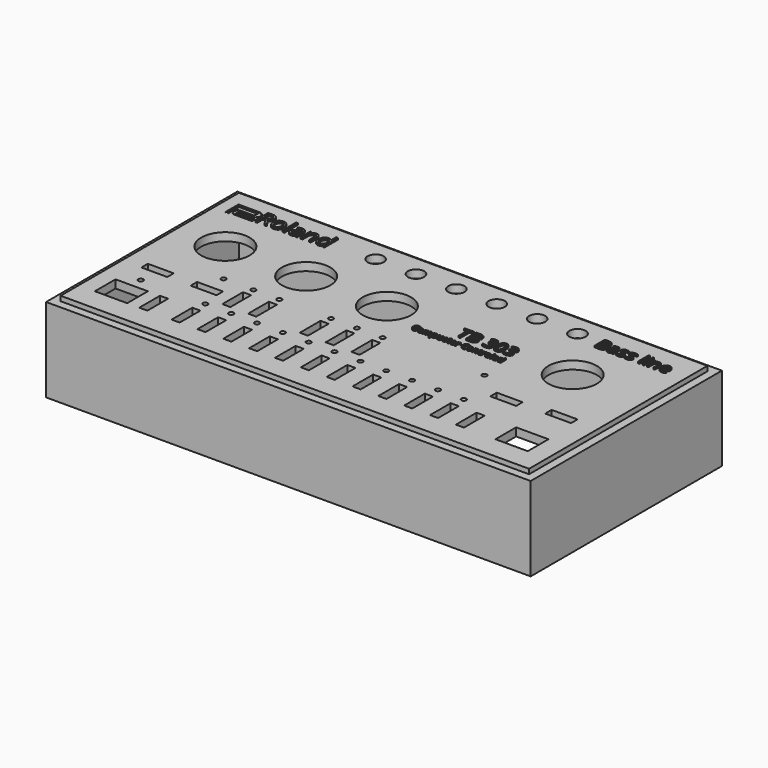
from build123d import *

# Parameters (mm, degrees)
F6_START       = 50
F0_W           = 290
F0_H           = 138
F6_DEPTH       = 5
F7_START       = 50
F4_W           = 5
F4_H           = 16
F4_W_2         = 20
F4_W_3         = 16
F4_H_2         = 5
F4_R           = 1.5
F3_R           = 15
F2_R           = 5
F7_DEPTH       = 5
F0_W_2         = 300
F0_H_2         = 148
F8_DEPTH       = 52
F9_START       = 55
F5_TEXT_SIZE   = 11.1111111111
F9_DEPTH       = 1
F10_START      = 55
F5_TEXT_SIZE_2 = 5.5555555556
F10_DEPTH      = 1
F11_START      = 55
F5_TEXT_SIZE_3 = 13.8888888889
F11_DEPTH      = 1
F12_START      = 55
F12_DEPTH      = 1
F15_W          = 0.5
F15_H          = 0.5


# Not quite as in the source:
# - a feature names something its author has since deleted; it is built from what else it names
# - Text() gives the source's letters only with a copy of the font that has no kerning and outlines rounded to 1/6400 em; it was checked with that copy


with BuildPart() as f6:
    # F0 (on Top) → F6 (new body)
    with BuildSketch(Plane.XY.offset(F6_START)):
        with Locations((150, 74)):
            Rectangle(F0_W, F0_H)
    extrude(amount=F6_DEPTH)

    # F4 (on Top) + F3 (on Top) + F2 (on Top) → F7 (cut)
    with BuildSketch(Plane.XY.offset(F7_START)):
        with Locations((161, 27)):
            Rectangle(F4_W, F4_H)
        with Locations((97, 27)):
            Rectangle(F4_W, F4_H)
        with Locations((241, 27)):
            Rectangle(F4_W, F4_H)
        with Locations((129, 27)):
            Rectangle(F4_W, F4_H)
        with Locations((113, 27)):
            Rectangle(F4_W, F4_H)
        with Locations((145, 27)):
            Rectangle(F4_W, F4_H)
        with Locations((177, 27)):
            Rectangle(F4_W, F4_H)
        with Locations((225, 27)):
            Rectangle(F4_W, F4_H)
        with Locations((25, 27)):
            Rectangle(F4_W_2, F4_H)
        with Locations((273, 27)):
            Rectangle(F4_W_2, F4_H)
        with Locations((209, 27)):
            Rectangle(F4_W, F4_H)
        with Locations((193, 27)):
            Rectangle(F4_W, F4_H)
        with Locations((273, 57.5)):
            Rectangle(F4_W_3, F4_H_2)
        with Locations((241, 55)):
            Rectangle(F4_W_3, F4_H_2)
        with Locations((65, 27)):
            Rectangle(F4_W, F4_H)
        with Locations((81, 27)):
            Rectangle(F4_W, F4_H)
        with Locations((138, 55)):
            Rectangle(F4_W, F4_H)
        with Locations((90, 55)):
            Rectangle(F4_W, F4_H)
        with Locations((74, 55)):
            Rectangle(F4_W, F4_H)
        with Locations((45, 27)):
            Rectangle(F4_W, F4_H)
        with Locations((25, 55)):
            Rectangle(F4_W_3, F4_H_2)
        with Locations((154, 55)):
            Rectangle(F4_W, F4_H)
        with Locations((122, 55)):
            Rectangle(F4_W, F4_H)
        with Locations((217, 68)):
            Circle(F4_R)
        with Locations((225, 42)):
            Circle(F4_R)
        with Locations((209, 42)):
            Circle(F4_R)
        with Locations((129, 42)):
            Circle(F4_R)
        with Locations((161, 42)):
            Circle(F4_R)
        with Locations((177, 42)):
            Circle(F4_R)
        with Locations((145, 42)):
            Circle(F4_R)
        with Locations((25, 42)):
            Circle(F4_R)
        with Locations((113, 42)):
            Circle(F4_R)
        with Locations((81, 42)):
            Circle(F4_R)
        with Locations((122, 68)):
            Circle(F4_R)
        with Locations((138, 68)):
            Circle(F4_R)
        with Locations((74, 68)):
            Circle(F4_R)
        with Locations((65, 42)):
            Circle(F4_R)
        with Locations((90, 68)):
            Circle(F4_R)
        with Locations((193, 42)):
            Circle(F4_R)
        with Locations((97, 42)):
            Circle(F4_R)
        with Locations((154, 68)):
            Circle(F4_R)
        with Locations((55.5, 55)):
            Rectangle(F4_W_3, F4_H_2)
        with Locations((55.5, 68)):
            Circle(F4_R)
    with BuildSketch(Plane.XY.offset(F7_START)):
        with Locations((250, 95)):
            Circle(F3_R)
        with Locations((85, 95)):
            Circle(F3_R)
        with Locations((35, 95)):
            Circle(F3_R)
        with Locations((135, 95)):
            Circle(F3_R)
    with BuildSketch(Plane.XY.offset(F7_START)):
        with Locations((200, 130)):
            Circle(F2_R)
        with Locations((175, 130)):
            Circle(F2_R)
        with Locations((150, 130)):
            Circle(F2_R)
        with Locations((100, 130)):
            Circle(F2_R)
        with Locations((125, 130)):
            Circle(F2_R)
        with Locations((225, 130)):
            Circle(F2_R)
    extrude(amount=F7_DEPTH, mode=Mode.SUBTRACT)

    # F0 (on Top) → F8 (join)
    with BuildSketch(Plane.XY):
        with Locations((150, 74)):
            Rectangle(F0_W_2, F0_H_2)
        with Locations((150, 74)):
            Rectangle(F0_W, F0_H, mode=Mode.SUBTRACT)
    extrude(amount=F8_DEPTH)

    # F5 (on Top) → F9 (join)
    with BuildSketch(Plane.XY.offset(F9_START)):
        with Locations((180.0296506865, 91)):
            Text('TB 303', F5_TEXT_SIZE, font='Open Sans', text_align=(TextAlign.LEFT, TextAlign.BOTTOM))
    extrude(amount=F9_DEPTH)

    # F5 (on Top) → F10 (join)
    with BuildSketch(Plane.XY.offset(F10_START)):
        with Locations((158.9749631865, 83)):
            Text('Compueter Controled', F5_TEXT_SIZE_2, font='Open Sans', text_align=(TextAlign.LEFT, TextAlign.BOTTOM))
    extrude(amount=F10_DEPTH)

    # F5 (on Top) → F11 (join)
    with BuildSketch(Plane.XY.offset(F11_START)):
        with Locations((29, 124)):
            Text('Roland', F5_TEXT_SIZE_3, font='Open Sans', text_align=(TextAlign.LEFT, TextAlign.BOTTOM))
    extrude(amount=F11_DEPTH)

    # F5 (on Top) → F12 (join)
    with BuildSketch(Plane.XY.offset(F12_START)):
        with Locations((239.3194444444, 124)):
            Text('Bass line', F5_TEXT_SIZE, font='Open Sans', text_align=(TextAlign.LEFT, TextAlign.BOTTOM))
    extrude(amount=F12_DEPTH)

    # F16: sweep along a path in F13
    with BuildLine(Plane.XY.offset(55)) as f16_path:
        Line((12.5535261929, 122.9964725018), (12.5535261929, 133.2))
        Line((12.5535261929, 133.2), (25.5535261929, 133.2))
        ThreePointArc((25.5535261929, 133.2), (28.5535261929, 130.2), (25.5535261929, 127.2))
        Line((25.5535261929, 127.2), (17.5535261929, 127.2))
        Line((17.5535261929, 127.2), (17.5535261929, 125.6))
        Line((17.5535261929, 125.6), (28.5535261929, 125.6))
    # F15 (on plane+point) → F16 (sweep)
    with BuildSketch(Plane.XZ.offset(-122.9964725018)):
        with Locations((12.5535261929, 55)):
            Rectangle(F15_W, F15_H)
    sweep(path=f16_path.line, transition=Transition.RIGHT)

    # F17: sweep along a path in F13
    with BuildLine(Plane.XY.offset(55)) as f17_path:
        Line((14.1535261929, 122.9964725018), (14.1535261929, 131.6))
        Line((14.1535261929, 131.6), (25.5535261929, 131.6))
        Line((25.5535261929, 131.6), (25.5535261929, 128.8))
        Line((25.5535261929, 128.8), (17.5535261929, 128.8))
        ThreePointArc((17.5535261929, 128.8), (15.1535261929, 126.4), (17.5535261929, 124))
        Line((17.5535261929, 124), (28.5535261929, 124))
    # F15 (on plane+point) → F17 (sweep)
    with BuildSketch(Plane.XZ.offset(-122.9964725018)):
        with Locations((14.1535261929, 55)):
            Rectangle(F15_W, F15_H)
    sweep(path=f17_path.line, transition=Transition.RIGHT)


solid = f6.part
